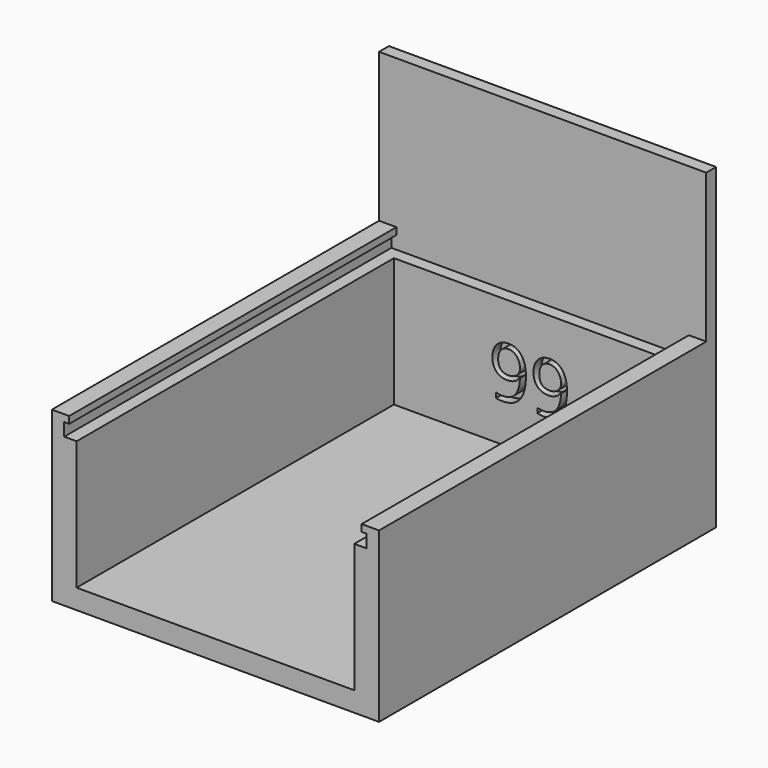
from build123d import *

# Parameters (mm, degrees)
F1_DEPTH     = 50.8
F0_W         = 71.12
F0_H         = 96.52
F2_DEPTH     = 12.7
F3_DEPTH     = 45.72
F4_W         = 99.695
F4_H         = 1.778
F5_DEPTH     = 1.27
F6_W         = 99.695
F6_H         = 1.778
F7_DEPTH     = 1.27
F8_TEXT_SIZE = 18.4131579267
F9_DEPTH     = 2.54
F10_W        = 83.82
F10_H        = 102.87
F11_DEPTH    = 7.62
F12_W        = 83.82
F12_H        = 3.175
F13_DEPTH    = 38.1
F15_DEPTH    = 5.08


# Not quite as in the source:
# - Text() gives the source's letters only with a copy of the font that has no kerning and outlines rounded to 1/6400 em; it was checked with that copy


with BuildPart() as f1:
    # F0 (on Top) → F1 (new body)
    with BuildSketch(Plane.XY):
        Polygon((-41.91, -42.5823529412), (-38.735, -42.5823529412), (-38.735, 57.1126470588), (38.735, 57.1126470588), (38.735, -42.5823529412), (41.91, -42.5823529412), (41.91, 60.2876470588), (-41.91, 60.2876470588), align=None)
    extrude(amount=F1_DEPTH)

    # F0 (on Top) → F2 (join)
    with BuildSketch(Plane.XY):
        with Locations((0, 5.6776470588)):
            Rectangle(F0_W, F0_H)
        Polygon((-35.56, -42.5823529412), (-35.56, 53.9376470588), (35.56, 53.9376470588), (35.56, -42.5823529412), (38.735, -42.5823529412), (38.735, 57.1126470588), (-38.735, 57.1126470588), (-38.735, -42.5823529412), align=None)
    extrude(amount=F2_DEPTH)

    # F0 (on Top) → F3 (join)
    with BuildSketch(Plane.XY):
        Polygon((-35.56, -42.5823529412), (-35.56, 53.9376470588), (35.56, 53.9376470588), (35.56, -42.5823529412), (38.735, -42.5823529412), (38.735, 57.1126470588), (-38.735, 57.1126470588), (-38.735, -42.5823529412), align=None)
    extrude(amount=F3_DEPTH)

    # F4 (on face) → F5 (join)
    with BuildSketch(Plane.YZ.offset(-38.735)):
        with Locations((7.2651470588, 49.911)):
            Rectangle(F4_W, F4_H)
    extrude(amount=F5_DEPTH)

    # F6 (on face) → F7 (join)
    with BuildSketch(Plane(origin=(38.735, 0, 0), x_dir=(0, -1, 0), z_dir=(-1, 0, 0))):
        with Locations((-7.2651470588, 49.911)):
            Rectangle(F6_W, F6_H)
    extrude(amount=F7_DEPTH)

    # F8 (on face) → F9 (cut)
    with BuildSketch(Plane.XZ.offset(-53.9376470588)):
        with Locations((-11.2804792006, 22.6772557944)):
            Text('99', F8_TEXT_SIZE, font='Open Sans', text_align=(TextAlign.LEFT, TextAlign.BOTTOM))
    extrude(amount=-F9_DEPTH, mode=Mode.SUBTRACT)

    # F10 (on face) → F11 (cut)
    with BuildSketch(Plane(origin=(0, 0, 0), x_dir=(1, 0, 0), z_dir=(0, 0, -1))):
        with Locations((0, -8.8526470588)):
            Rectangle(F10_W, F10_H)
    extrude(amount=-F11_DEPTH, mode=Mode.SUBTRACT)

    # F12 (on face) → F13 (join)
    with BuildSketch(Plane.XY.offset(50.8)):
        with Locations((0, 58.7001470588)):
            Rectangle(F12_W, F12_H)
    extrude(amount=F13_DEPTH)

    # F14 (on face) → F15 (join)
    with BuildSketch(Plane.XZ.offset(42.5823529412)):
        Polygon((-37.465, 49.022), (-37.465, 50.8), (-41.91, 50.8), (-41.91, 7.62), (41.91, 7.62), (41.91, 50.8), (37.465, 50.8), (37.465, 49.022), (38.735, 49.022), (38.735, 45.72), (35.56, 45.72), (35.56, 12.7), (-35.56, 12.7), (-35.56, 45.72), (-38.735, 45.72), (-38.735, 49.022), align=None)
    extrude(amount=F15_DEPTH)


solid = f1.part
